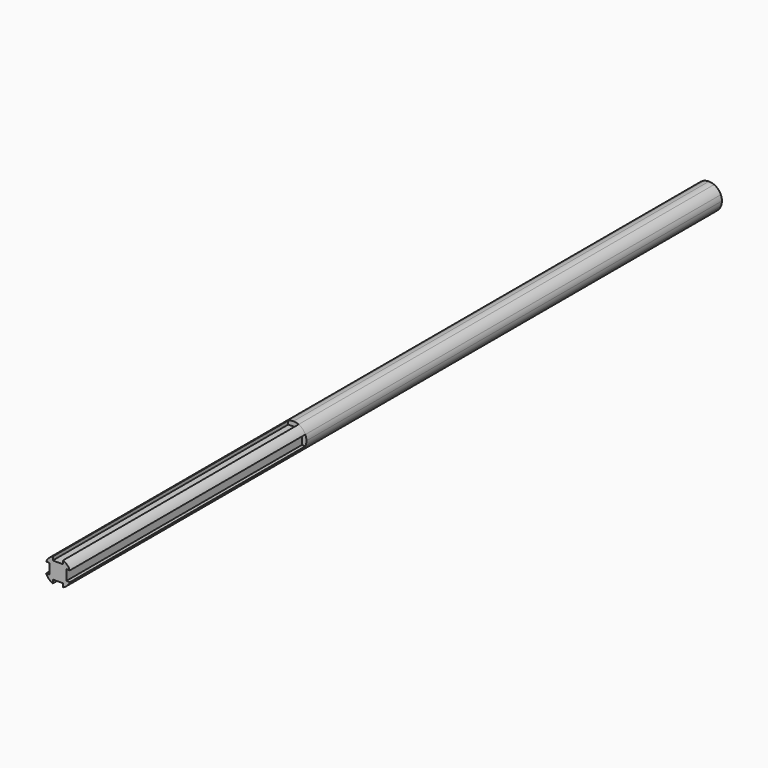
from build123d import *
from build123d import SkipClean  # not in build123d's __all__

# Parameters (mm, degrees)
F1_DEPTH = 51
F2_DEPTH = 90


with BuildPart() as f1:
    # F0 (on Front) → F1 (new body)
    with BuildSketch(Plane.XZ):
        with BuildLine():
            Line((1.45, 0.9), (2.0621590627, 0.9))
            ThreePointArc((2.0621590627, 0.9), (1.5909902577, 1.5909902577), (0.9, 2.0621590627))
            Line((0.9, 2.0621590627), (0.9, 1.45))
            Line((0.9, 1.45), (0, 1.45))
            Line((0, 1.45), (-0.9, 1.45))
            Line((-0.9, 1.45), (-0.9, 2.0621590627))
            ThreePointArc((-0.9, 2.0621590627), (-1.5909902577, 1.5909902577), (-2.0621590627, 0.9))
            Line((-2.0621590627, 0.9), (-1.45, 0.9))
            Line((-1.45, 0.9), (-1.45, 0))
            Line((-1.45, 0), (-1.45, -0.9))
            Line((-1.45, -0.9), (-2.0621590627, -0.9))
            ThreePointArc((-2.0621590627, -0.9), (-1.5909902577, -1.5909902577), (-0.9, -2.0621590627))
            Line((-0.9, -2.0621590627), (-0.9, -1.45))
            Line((-0.9, -1.45), (0, -1.45))
            Line((0, -1.45), (0.9, -1.45))
            Line((0.9, -1.45), (0.9, -2.0621590627))
            ThreePointArc((0.9, -2.0621590627), (1.5909902577, -1.5909902577), (2.0621590627, -0.9))
            Line((2.0621590627, -0.9), (1.45, -0.9))
            Line((1.45, -0.9), (1.45, 0))
            Line((1.45, 0), (1.45, 0.9))
        make_face()
    extrude(amount=F1_DEPTH)

    # F0 (on Front) → F2 (join)
    with BuildSketch(Plane.XZ):
        with BuildLine():
            Line((1.45, 0.9), (2.0621590627, 0.9))
            ThreePointArc((2.0621590627, 0.9), (1.5909902577, 1.5909902577), (0.9, 2.0621590627))
            Line((0.9, 2.0621590627), (0.9, 1.45))
            Line((0.9, 1.45), (0, 1.45))
            Line((0, 1.45), (-0.9, 1.45))
            Line((-0.9, 1.45), (-0.9, 2.0621590627))
            ThreePointArc((-0.9, 2.0621590627), (-1.5909902577, 1.5909902577), (-2.0621590627, 0.9))
            Line((-2.0621590627, 0.9), (-1.45, 0.9))
            Line((-1.45, 0.9), (-1.45, 0))
            Line((-1.45, 0), (-1.45, -0.9))
            Line((-1.45, -0.9), (-2.0621590627, -0.9))
            ThreePointArc((-2.0621590627, -0.9), (-1.5909902577, -1.5909902577), (-0.9, -2.0621590627))
            Line((-0.9, -2.0621590627), (-0.9, -1.45))
            Line((-0.9, -1.45), (0, -1.45))
            Line((0, -1.45), (0.9, -1.45))
            Line((0.9, -1.45), (0.9, -2.0621590627))
            ThreePointArc((0.9, -2.0621590627), (1.5909902577, -1.5909902577), (2.0621590627, -0.9))
            Line((2.0621590627, -0.9), (1.45, -0.9))
            Line((1.45, -0.9), (1.45, 0))
            Line((1.45, 0), (1.45, 0.9))
        make_face()
        with BuildLine():
            Line((0.9, 1.45), (0.9, 2.0621590627))
            ThreePointArc((0.9, 2.0621590627), (0.4596966983, 2.2025392041), (0, 2.25))
            ThreePointArc((0, 2.25), (-0.4596966983, 2.2025392041), (-0.9, 2.0621590627))
            Line((-0.9, 2.0621590627), (-0.9, 1.45))
            Line((-0.9, 1.45), (0, 1.45))
            Line((0, 1.45), (0.9, 1.45))
        make_face()
        with BuildLine():
            Line((-1.45, 0.9), (-2.0621590627, 0.9))
            ThreePointArc((-2.0621590627, 0.9), (-2.2025392041, 0.4596966983), (-2.25, 0))
            ThreePointArc((-2.25, 0), (-2.2025392041, -0.4596966983), (-2.0621590627, -0.9))
            Line((-2.0621590627, -0.9), (-1.45, -0.9))
            Line((-1.45, -0.9), (-1.45, 0))
            Line((-1.45, 0), (-1.45, 0.9))
        make_face()
        with BuildLine():
            ThreePointArc((0, -2.25), (0.4596966983, -2.2025392041), (0.9, -2.0621590627))
            Line((0.9, -2.0621590627), (0.9, -1.45))
            Line((0.9, -1.45), (0, -1.45))
            Line((0, -1.45), (-0.9, -1.45))
            Line((-0.9, -1.45), (-0.9, -2.0621590627))
            ThreePointArc((-0.9, -2.0621590627), (-0.4596966983, -2.2025392041), (0, -2.25))
        make_face()
        with BuildLine():
            ThreePointArc((2.0621590627, -0.9), (2.2025392041, -0.4596966983), (2.25, 0))
            ThreePointArc((2.25, 0), (2.2025392041, 0.4596966983), (2.0621590627, 0.9))
            Line((2.0621590627, 0.9), (1.45, 0.9))
            Line((1.45, 0.9), (1.45, 0))
            Line((1.45, 0), (1.45, -0.9))
            Line((1.45, -0.9), (2.0621590627, -0.9))
        make_face()
    with SkipClean():  # cleaning this boolean's faces spoils the solid; the shape is the same uncleaned
        extrude(amount=-F2_DEPTH)


solid = f1.part
